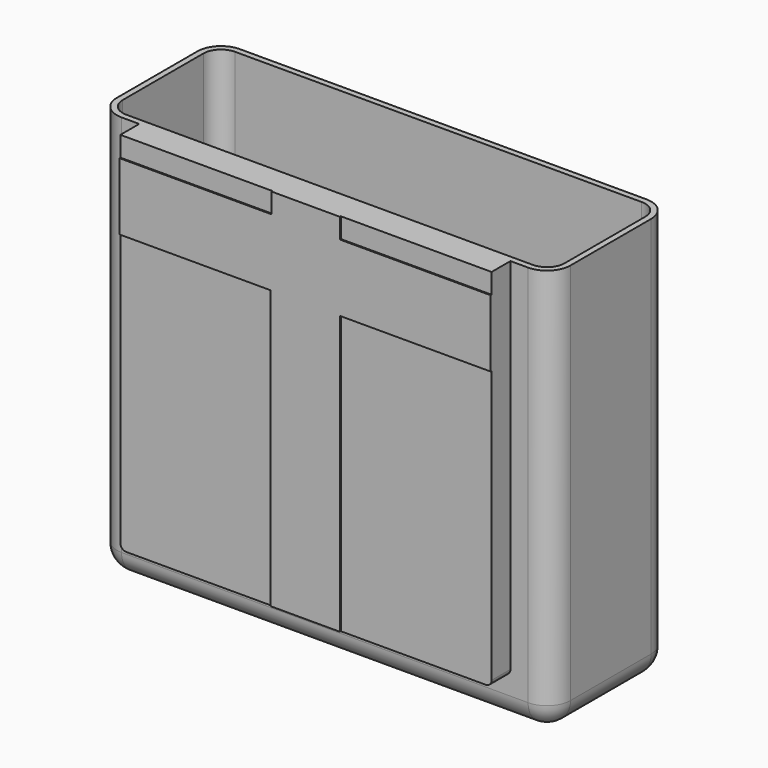
from build123d import *

# Parameters (mm, degrees)
F1_DEPTH     = 12.55
F2_R         = 2
F3_T1_DEPTH  = 37.5
F3_T3_DEPTH  = 8.55
F3_T5_DEPTH  = 34.5
F3_S9_W      = 2
F3_S9_H      = 2
F3_T10_DEPTH = 2
F3_S15_W     = 2
F3_S15_H     = 2
F3_T16_DEPTH = 2
F3_S21_W     = 2
F3_S21_H     = 2
F3_T22_DEPTH = 2
F3_S27_W     = 2
F3_S27_H     = 2
F3_T28_DEPTH = 2
F4_T         = -0.5
F6_W         = 31.5
F6_H         = 31
F7_DEPTH     = 2
F8_R         = 0.5
F10_DEPTH    = 0.1


# Not quite as in the source:
# - a fillet or chamfer that OpenCascade refuses, or shapes differently, is made with other operations: its cross-section is extruded or revolved along the edge and cut away or added


with BuildPart() as f1:
    # F0 (on Front) → F1 (new body)
    with BuildSketch(Plane.XZ):
        Polygon((-42.1370128049, 10.5798164573), (-42.1370128049, -23.9201835427), (-3.6370128049, -23.9201835427), (-3.6370128049, 10.5798164573), (-8.2607226698, 10.5798164573), (-39.5151264966, 10.5798164573), (-39.6370128049, 10.5798164573), align=None)
    extrude(amount=F1_DEPTH)

    # F2
    f2_edges = [f1.edges().sort_by_distance(p)[0] for p in [
        (-42.137013, -12.55, -6.670184),
        (-22.887013, -12.55, -23.920184),
        (-3.637013, -12.55, -6.670184),
    ]]
    fillet(f2_edges, radius=F2_R)

    # F3: fillet of radius 2 on 5 edges, made by hand

    # F3_s2 → F3_t1 (cut)
    with BuildSketch(Plane.XY.offset(-21.9201835427)):
        with BuildLine():
            ThreePointArc((-42.1370128049, -2), (-41.5512263672, -0.5857864376), (-40.1370128049, 0))
            Line((-40.1370128049, 0), (-42.1370128049, 0))
            Line((-42.1370128049, 0), (-42.1370128049, -2))
        make_face()
        with BuildLine():
            ThreePointArc((-5.6370128049, 0), (-4.2227992425, -0.5857864376), (-3.6370128049, -2))
            Line((-3.6370128049, -2), (-3.6370128049, 0))
            Line((-3.6370128049, 0), (-5.6370128049, 0))
        make_face()
    extrude(amount=F3_T1_DEPTH, mode=Mode.SUBTRACT)

    # F3_s4 → F3_t3 (cut)
    with BuildSketch(Plane.XZ.offset(2)):
        with BuildLine():
            ThreePointArc((-5.6370128049, -23.9201835427), (-4.2227992425, -23.3343971051), (-3.6370128049, -21.9201835427))
            Line((-3.6370128049, -21.9201835427), (-3.6370128049, -23.9201835427))
            Line((-3.6370128049, -23.9201835427), (-5.6370128049, -23.9201835427))
        make_face()
        with BuildLine():
            ThreePointArc((-42.1370128049, -21.9201835427), (-41.5512263672, -23.3343971051), (-40.1370128049, -23.9201835427))
            Line((-40.1370128049, -23.9201835427), (-42.1370128049, -23.9201835427))
            Line((-42.1370128049, -23.9201835427), (-42.1370128049, -21.9201835427))
        make_face()
    extrude(amount=F3_T3_DEPTH, mode=Mode.SUBTRACT)

    # F3_s6 → F3_t5 (cut)
    with BuildSketch(Plane.YZ.offset(-40.1370128049)):
        with BuildLine():
            ThreePointArc((0, -21.9201835427), (-0.5857864376, -23.3343971051), (-2, -23.9201835427))
            Line((-2, -23.9201835427), (0, -23.9201835427))
            Line((0, -23.9201835427), (0, -21.9201835427))
        make_face()
    extrude(amount=F3_T5_DEPTH, mode=Mode.SUBTRACT)


with BuildPart() as f3_tool8:
    # F3_s9 → F3_t10 (new body)
    with BuildSketch(Plane.YZ.offset(-40.1370128049)):
        with Locations((-11.55, -22.9201835427)):
            Rectangle(F3_S9_W, F3_S9_H)
    extrude(amount=-F3_T10_DEPTH)

    # F3_s11 → F3_t12 (revolve, cut)
    with BuildSketch(Plane(origin=(-40.1370128049, -10.55, -21.9201835427), x_dir=(0, 0.7071067812, 0.7071067812), z_dir=(0, -0.7071067812, 0.7071067812))):
        with BuildLine():
            ThreePointArc((0, -2), (2, 0), (0, 2))
            Line((0, 2), (0, -2))
        make_face()
    revolve(axis=Axis((-40.1370128049, -10.55, -21.9201835427), (-1, 0, 0)), mode=Mode.SUBTRACT)


with BuildPart() as f1_1:
    add(f1.part)

    # F3_t7: cut F3_tool8
    add(f3_tool8.part, mode=Mode.SUBTRACT)


with BuildPart() as f3_tool14:
    # F3_s15 → F3_t16 (new body)
    with BuildSketch(Plane.XY.offset(-21.9201835427)):
        with Locations((-4.6370128049, -11.55)):
            Rectangle(F3_S15_W, F3_S15_H)
    extrude(amount=-F3_T16_DEPTH)

    # F3_s17 → F3_t18 (revolve, cut)
    with BuildSketch(Plane(origin=(-5.6370128049, -10.55, -21.9201835427), x_dir=(-0.7071067812, 0.7071067812, 0), z_dir=(-0.7071067812, -0.7071067812, 0))):
        with BuildLine():
            ThreePointArc((0, -2), (2, 0), (0, 2))
            Line((0, 2), (0, -2))
        make_face()
    revolve(axis=Axis((-5.6370128049, -10.55, -21.9201835427), (0, 0, -1)), mode=Mode.SUBTRACT)


with BuildPart() as f1_2:
    add(f1_1.part)

    # F3_t13: cut F3_tool14
    add(f3_tool14.part, mode=Mode.SUBTRACT)


with BuildPart() as f3_tool20:
    # F3_s21 → F3_t22 (new body)
    with BuildSketch(Plane.YZ.offset(-40.1370128049)):
        with Locations((-1, -22.9201835427)):
            Rectangle(F3_S21_W, F3_S21_H)
    extrude(amount=-F3_T22_DEPTH)

    # F3_s23 → F3_t24 (revolve, cut)
    with BuildSketch(Plane(origin=(-40.1370128049, -2, -21.9201835427), x_dir=(0, -0.7071067812, 0.7071067812), z_dir=(0, -0.7071067812, -0.7071067812))):
        with BuildLine():
            ThreePointArc((0, -2), (2, 0), (0, 2))
            Line((0, 2), (0, -2))
        make_face()
    revolve(axis=Axis((-40.1370128049, -2, -21.9201835427), (-1, 0, 0)), mode=Mode.SUBTRACT)


with BuildPart() as f1_3:
    add(f1_2.part)

    # F3_t19: cut F3_tool20
    add(f3_tool20.part, mode=Mode.SUBTRACT)


with BuildPart() as f3_tool26:
    # F3_s27 → F3_t28 (new body)
    with BuildSketch(Plane.XZ.offset(2)):
        with Locations((-4.6370128049, -22.9201835427)):
            Rectangle(F3_S27_W, F3_S27_H)
    extrude(amount=-F3_T28_DEPTH)

    # F3_s29 → F3_t30 (revolve, cut)
    with BuildSketch(Plane(origin=(-5.6370128049, -2, -21.9201835427), x_dir=(-0.7071067812, 0, 0.7071067812), z_dir=(-0.7071067812, 0, -0.7071067812))):
        with BuildLine():
            ThreePointArc((0, -2), (2, 0), (0, 2))
            Line((0, 2), (0, -2))
        make_face()
    revolve(axis=Axis((-5.6370128049, -2, -21.9201835427), (0, 1, 0)), mode=Mode.SUBTRACT)


with BuildPart() as f1_4:
    add(f1_3.part)

    # F3_t25: cut F3_tool26
    add(f3_tool26.part, mode=Mode.SUBTRACT)

    # F4
    f4_openings = [f1_4.faces().sort_by_distance(p)[0] for p in [
        (-22.887013, -6.275, 10.579816),
    ]]
    offset(amount=F4_T, openings=f4_openings)

    # F6 (on offset) → F7 (join)
    with BuildSketch(Plane.XZ.offset(12.55)):
        with Locations((-22.8870128049, -4.9201835427)):
            Rectangle(F6_W, F6_H)
    extrude(amount=F7_DEPTH)

    # F8
    f8_edges = [f1_4.edges().sort_by_distance(p)[0] for p in [
        (-38.637013, -13.55, -20.420184),
        (-7.137013, -13.55, -20.420184),
    ]]
    fillet(f8_edges, radius=F8_R)

    # F9 (on face) → F10 (join)
    with BuildSketch(Plane.XZ.offset(14.55)):
        Polygon((-25.7187689085, 8.8785898675), (-38.6370128049, 8.8785898675), (-38.6370128049, 3.1798164573), (-25.8370128049, 3.1798164573), (-25.8370128049, -20.4201835427), (-19.9370128049, -20.4201835427), (-19.9370128049, 3.1798164573), (-7.1370128049, 3.1798164573), (-7.1370128049, 8.8798164573), (-19.9370128049, 8.8798164573), (-19.9370128049, 10.5798164573), (-25.7187689085, 10.5798164573), align=None)
    extrude(amount=F10_DEPTH)


solid = f1_4.part
